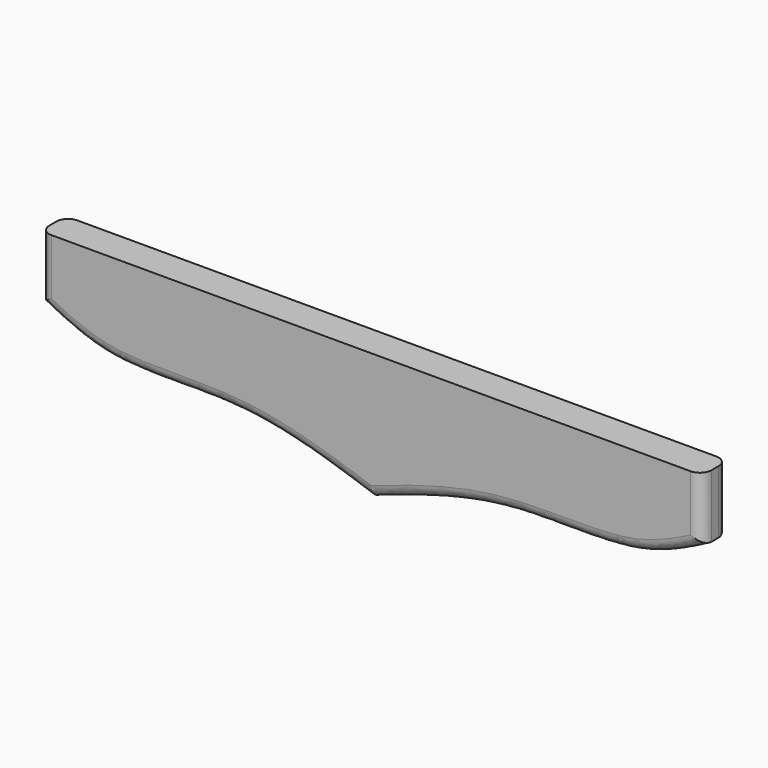
from build123d import *

# Parameters (mm, degrees)
F0_W     = 65.5089840293
F0_H     = 12.4657871202
F1_DEPTH = 3.175
F2_R     = 2.286


with BuildPart() as f1:
    # F0 (on Front) → F1 (new body, symmetric)
    with BuildSketch(Plane.XZ):
        with Locations((32.7544920146, 6.2328935601)):
            Rectangle(F0_W, F0_H)
        with Locations((-32.7544920146, 6.2328935601)):
            Rectangle(F0_W, F0_H)
        with BuildLine():
            Line((65.5089840293, 0), (0, 0))
            Line((0, 0), (0, -12.9745937884))
            add(Edge.make_bspline(
                [(0, -12.9745937884), (8.4051395557, -10.1107367384), (25.0248568997, -4.4479521566), (51.2725717155, -7.3050479768), (61.1865127872, -2.2179646884), (65.5089840293, 0)],
                knots=[0, 0, 0, 0, 0.3659185269, 0.7235409296, 1, 1, 1, 1], degree=3))
        make_face()
        with BuildLine():
            Line((0, -12.9745937884), (0, 0))
            Line((0, 0), (-65.5089840293, 0))
            add(Edge.make_bspline(
                [(0, -12.9745937884), (-8.4051395557, -10.1107367384), (-25.0248568997, -4.4479521566), (-51.2725717155, -7.3050479768), (-61.1865127872, -2.2179646884), (-65.5089840293, 0)],
                knots=[0, 0, 0, 0, 0.3659185269, 0.7235409296, 1, 1, 1, 1], degree=3))
        make_face()
    extrude(amount=F1_DEPTH, both=True)

    # F2
    f2_edges = [f1.edges().sort_by_distance(p)[0] for p in [
        (-32.834886, -3.175, -5.993997),
        (32.834886, -3.175, -5.993997),
        (32.834886, 3.175, -5.993997),
        (-32.834886, 3.175, -5.993997),
        (65.508984, 3.175, 6.232894),
        (65.508984, -3.175, 6.232894),
        (-65.508984, 3.175, 6.232894),
        (-65.508984, -3.175, 6.232894),
    ]]
    fillet(f2_edges, radius=F2_R)


solid = f1.part
